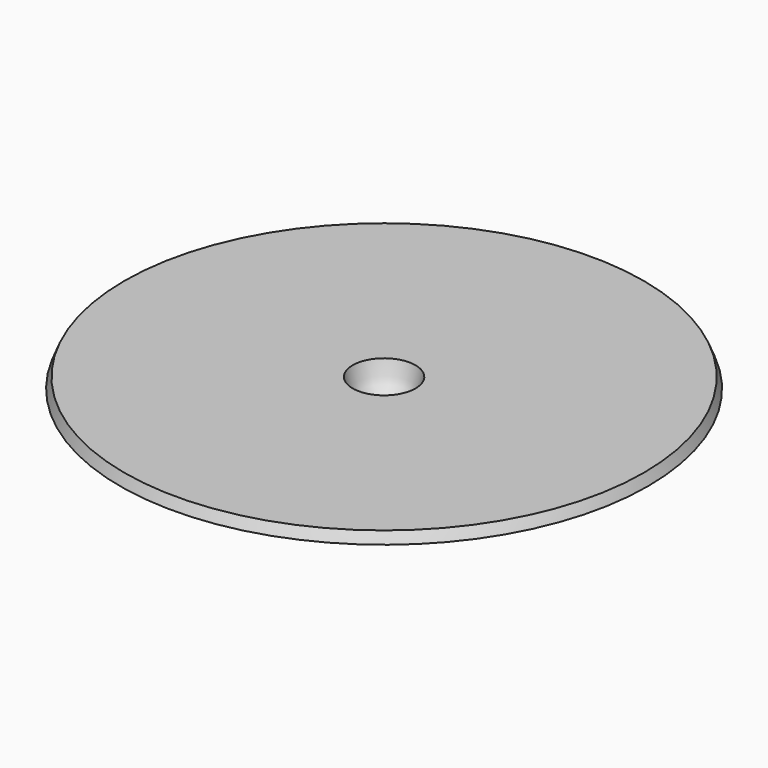
from build123d import *


with BuildPart() as f1:
    # F0 (on Front) → F1 (revolve)
    with BuildSketch(Plane.XZ):
        with BuildLine():
            ThreePointArc((15.875, -11.2468861043), (19.5966413277, -6.152735897), (20.9912098944, 0))
            Line((20.9912098944, 0), (160.02, 0))
            Line((160.02, 0), (157.48, 6.35))
            Line((157.48, 6.35), (19.05, 6.35))
            add(Edge.make_bspline(
                [(19.05, 6.35), (17.2943395607, -5.2739201542), (10.3896663187, -7.9876436539), (9.4300154597, -16.612906009), (9.525, -23.8922853023)],
                knots=[0, 0, 0, 0, 0.5270987441, 1, 1, 1, 1], degree=3))
            Line((9.525, -23.8922853023), (9.525, -40.0551594794))
            add(Edge.make_bspline(
                [(15.875, -50.8), (14.4695304334, -45.8264946938), (9.4677070156, -44.9470542371), (9.525, -40.0551594794)],
                knots=[0, 0, 0, 0, 12.4809493955, 12.4809493955, 12.4809493955, 12.4809493955], degree=3))
            Line((15.875, -50.8), (15.875, -11.2468861043))
        make_face()
    revolve(axis=Axis((0, 0, 2.4035767974), (0, 0, -1)))


solid = f1.part
